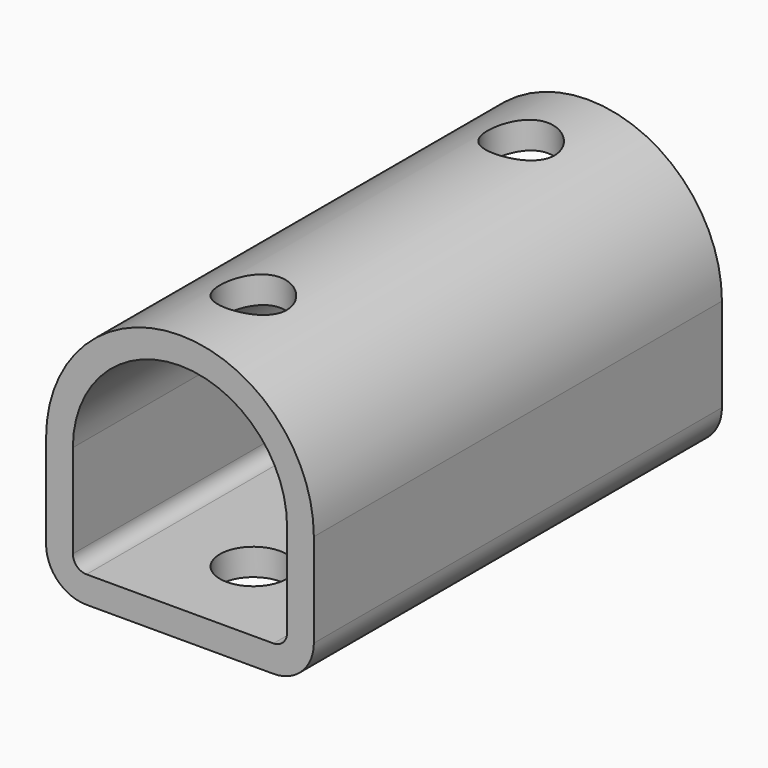
from build123d import *

# Parameters (mm, degrees)
F1_DEPTH      = 76.2
F2_R          = 4.99999
F3_DEPTH      = 20.00096
F3_DEPTH_BACK = 25.4


with BuildPart() as f1:
    # F0 (on Front) → F1 (new body)
    with BuildSketch(Plane.XZ):
        with BuildLine():
            ThreePointArc((19.99996, 0), (0, 19.99996), (-19.99996, 0))
            Line((-19.99996, 0), (-19.99996, -14.00556))
            ThreePointArc((-19.99996, -14.00556), (-18.2442408891, -18.2442408891), (-14.00556, -19.99996))
            Line((-14.00556, -19.99996), (14.00556, -19.99996))
            ThreePointArc((14.00556, -19.99996), (18.2442408891, -18.2442408891), (19.99996, -14.00556))
            Line((19.99996, -14.00556), (19.99996, 0))
        make_face()
        with BuildLine():
            Line((-15.99946, -13.96746), (-15.99946, 0))
            ThreePointArc((-15.99946, 0), (0, 15.99946), (15.99946, 0))
            Line((15.99946, 0), (15.99946, -13.96746))
            ThreePointArc((15.99946, -13.96746), (15.4043009794, -15.4043009794), (13.96746, -15.99946))
            Line((13.96746, -15.99946), (-13.96746, -15.99946))
            ThreePointArc((-13.96746, -15.99946), (-15.4043009794, -15.4043009794), (-15.99946, -13.96746))
        make_face(mode=Mode.SUBTRACT)
    extrude(amount=F1_DEPTH)

    # F2 (on Top) → F3 (cut, two sides)
    with BuildSketch(Plane.XY) as f3_sk:
        with Locations((0, -62.4967)):
            Circle(F2_R)
        with Locations((0, -12.4968)):
            Circle(F2_R)
    extrude(amount=-F3_DEPTH, mode=Mode.SUBTRACT)
    extrude(f3_sk.sketch, amount=F3_DEPTH_BACK, mode=Mode.SUBTRACT)


solid = f1.part
